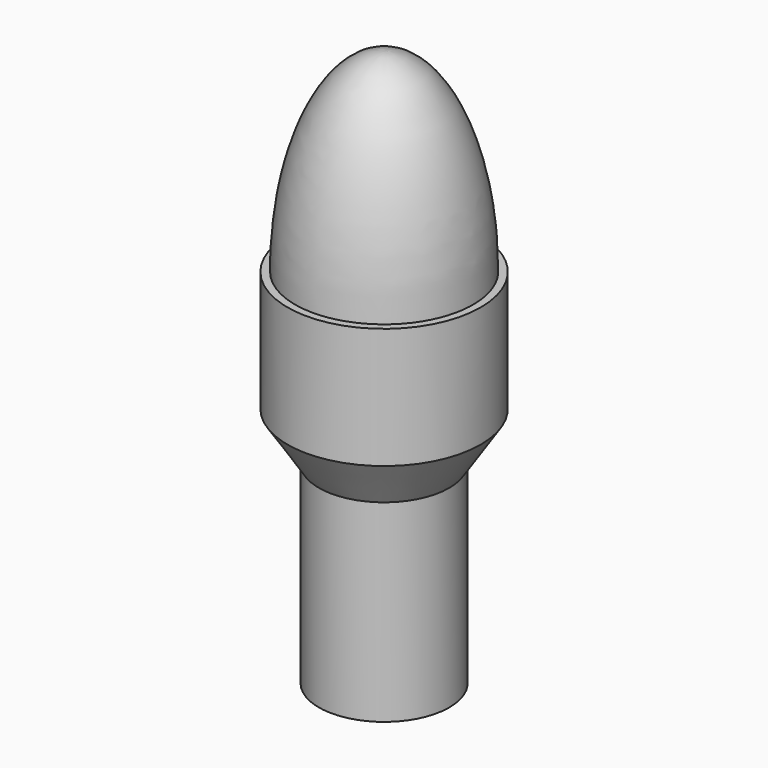
from build123d import *

# Parameters (mm, degrees)
F0_R      = 13.5
F1_DEPTH  = 40
F1_FACE_R = 13.5
F2_DEPTH  = 10
F2_TAPER  = -33.02
F3_DEPTH  = 25


with BuildPart() as f1:
    # F0 (on Top) → F1 (new body)
    with BuildSketch(Plane.XY):
        Circle(F0_R)
    extrude(amount=F1_DEPTH)

    # F1_face (on face) → F2 (join)
    with BuildSketch(Plane.XY.offset(40)):
        Circle(F1_FACE_R)
    extrude(amount=F2_DEPTH, taper=F2_TAPER)

    # F3 (add): a face of the model
    f3_faces = [f1.faces().sort_by_distance(p)[0] for p in [
        (0, 0, 50),
    ]]
    extrude(f3_faces, amount=F3_DEPTH)

    # F4 (on Right) → F5 (revolve)
    with BuildSketch(Plane.YZ):
        with BuildLine():
            add(Edge.make_bspline(
                [(0, 115), (-18.4366899531, 115), (-18.4366899531, 75.3298997879), (-18.4366899531, 35.6597995758), (0, 35.6597995758)],
                knots=[0, 0, 0, 1.5707963268, 1.5707963268, 3.1415926536, 3.1415926536, 3.1415926536], degree=2, weights=[1, 0.7071067812, 1, 0.7071067812, 1]))
            Line((0, 35.6597995758), (0, 115))
        make_face()
    revolve(axis=Axis((0, 0, 57.5), (0, 0, 1)))


solid = f1.part
